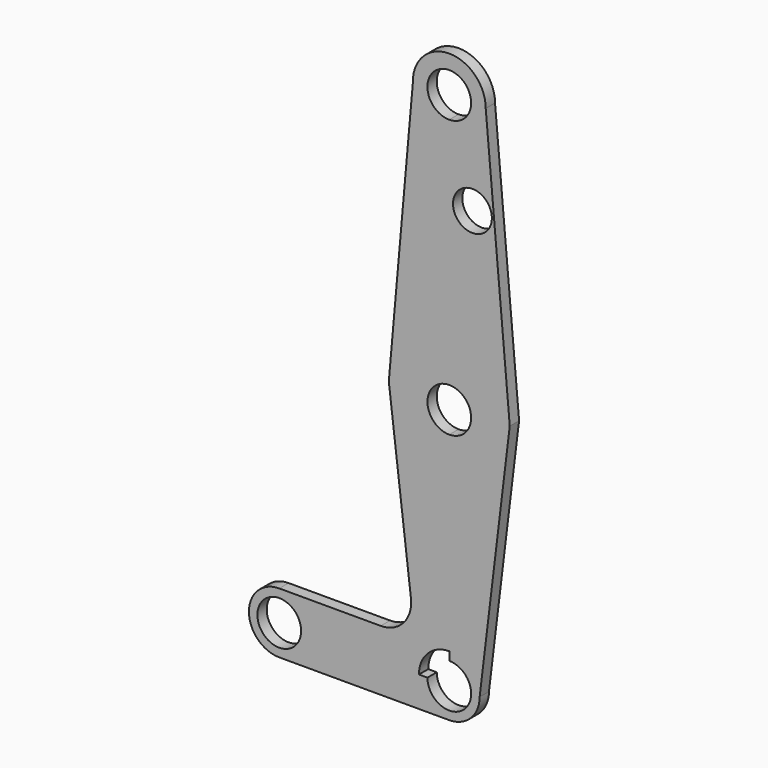
from build123d import *

# Parameters (mm, degrees)
F0_R     = 5.08
F0_R_2   = 5.715
F1_DEPTH = 3.048


# Not quite as in the source:
# - a feature of the source that left no trace in its solid (it failed there, or was rolled back) is left out


with BuildPart() as f1:
    # F0 (on Front) → F1 (new body)
    with BuildSketch(Plane.XZ):
        with BuildLine():
            ThreePointArc((0, 57.785), (-5.715, 63.5), (0, 69.215))
            Line((0, 69.215), (0, 126.4542473564))
            ThreePointArc((0, 126.4542473564), (-6.6367069731, 129.1469896364), (-9.5209852919, 135.7027259805))
            Line((-9.5209852919, 135.7027259805), (-15.8126809955, 64.9052561096))
            Line((-15.8126809955, 64.9052561096), (-10.0230526485, 16.8384262865))
            ThreePointArc((-10.0230526485, 16.8384262865), (-11.9679184287, 10.6128911922), (-17.9162015492, 7.9375))
            Line((-17.9162015492, 7.9375), (-44.45, 7.9375))
            ThreePointArc((-44.45, 7.9375), (-38.8373399243, 5.6126600757), (-36.5125, 0))
            Line((-36.5125, 0), (-7.9375, 0))
            ThreePointArc((-7.9375, 0), (-5.6126600757, 5.6126600757), (0, 7.9375))
            Line((0, 7.9375), (0, 57.785))
        make_face()
        with BuildLine():
            Line((0, 126.4542473564), (0, 69.215))
            ThreePointArc((0, 69.215), (4.0411152545, 67.5411152545), (5.715, 63.5))
            ThreePointArc((5.715, 63.5), (4.0411152545, 59.4588847455), (0, 57.785))
            Line((0, 57.785), (0, 7.9375))
            ThreePointArc((0, 7.9375), (5.6126600757, 5.6126600757), (7.9375, 0))
            Line((7.9375, 0), (15.8132155809, 64.8992276415))
            Line((15.8132155809, 64.8992276415), (9.5249892223, 135.9649185116))
            ThreePointArc((9.5249892223, 135.9649185116), (6.7301241724, 129.2389911578), (0, 126.4542473564))
        make_face()
        with Locations((6.0517773964, 111.243724823)):
            Circle(F0_R, mode=Mode.SUBTRACT)
        with BuildLine():
            ThreePointArc((-9.5209852919, 135.7027259805), (-6.6367069731, 129.1469896364), (0, 126.4542473564))
            ThreePointArc((0, 126.4542473564), (6.7301241724, 129.2389911578), (9.5249892223, 135.9649185116))
            ThreePointArc((9.5249892223, 135.9649185116), (9.5249973056, 135.972082932), (9.525, 135.9792473564))
            ThreePointArc((9.525, 135.9792473564), (-0.1382752592, 145.5032436265), (-9.5209852919, 135.7027259805))
        make_face()
        with BuildLine():
            ThreePointArc((5.715, 135.9792473564), (4.0411152545, 131.9381321019), (0, 130.2642473564))
            ThreePointArc((0, 130.2642473564), (-4.0411152545, 140.0203626109), (5.715, 135.9792473564))
        make_face(mode=Mode.SUBTRACT)
        with BuildLine():
            ThreePointArc((7.9375, 0), (5.6126600757, 5.6126600757), (0, 7.9375))
            Line((0, 7.9375), (0, 5.715))
            ThreePointArc((0, 5.715), (4.0411152545, 4.0411152545), (5.715, 0))
            ThreePointArc((5.715, 0), (0, -5.715), (-5.715, 0))
            Line((-5.715, 0), (-7.9375, 0))
            ThreePointArc((-7.9375, 0), (-5.6126600757, -5.6126600757), (0, -7.9375))
            ThreePointArc((0, -7.9375), (5.6126600757, -5.6126600757), (7.9375, 0))
        make_face()
        with BuildLine():
            ThreePointArc((0, -7.9375), (-5.6126600757, -5.6126600757), (-7.9375, 0))
            Line((-7.9375, 0), (-36.5125, 0))
            ThreePointArc((-36.5125, 0), (-38.8373399243, -5.6126600757), (-44.45, -7.9375))
            Line((-44.45, -7.9375), (0, -7.9375))
        make_face()
        with BuildLine():
            ThreePointArc((-44.45, -7.9375), (-38.8373399243, -5.6126600757), (-36.5125, 0))
            ThreePointArc((-36.5125, 0), (-38.8373399243, 5.6126600757), (-44.45, 7.9375))
            ThreePointArc((-44.45, 7.9375), (-52.3875, 0), (-44.45, -7.9375))
        make_face()
        with Locations((-44.45, 0)):
            Circle(F0_R_2, mode=Mode.SUBTRACT)
    extrude(amount=F1_DEPTH)


solid = f1.part
